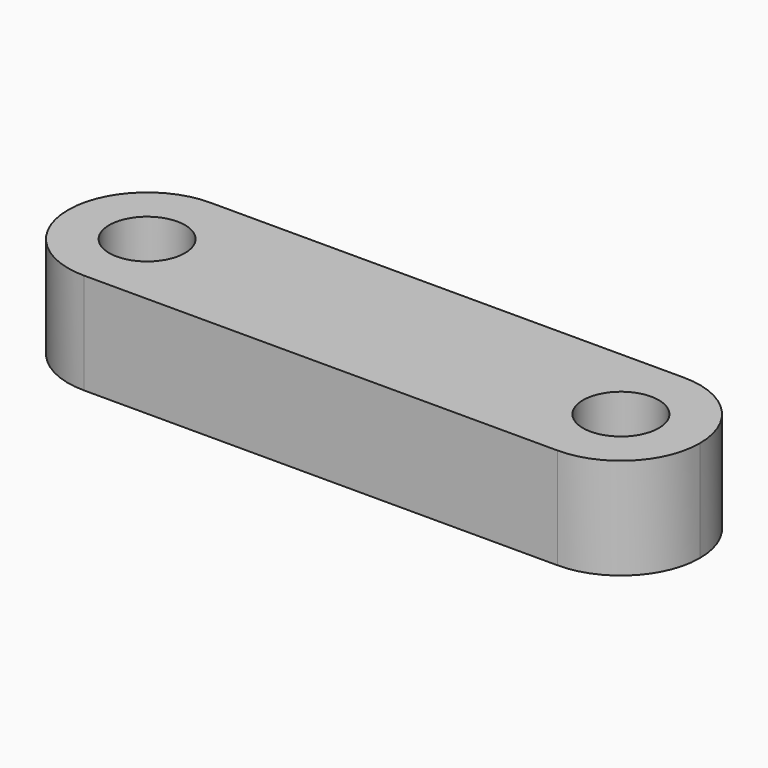
from build123d import *

# Parameters (mm, degrees)
F0_R     = 6
F1_DEPTH = 16


# Not quite as in the source:
# - a feature names something its author has since deleted; it is built from what else it names


with BuildPart() as f1:
    # F0 (on Top) → F1 (new body)
    with BuildSketch(Plane.XY):
        with BuildLine():
            Line((75, 12.5), (0, 12.5))
            ThreePointArc((0, 12.5), (8.8388347648, 8.8388347648), (12.5, 0))
            ThreePointArc((12.5, 0), (8.8388347648, -8.8388347648), (0, -12.5))
            Line((0, -12.5), (75, -12.5))
            ThreePointArc((75, -12.5), (62.5, 0), (75, 12.5))
        make_face()
        with BuildLine():
            ThreePointArc((12.5, 0), (8.8388347648, 8.8388347648), (0, 12.5))
            ThreePointArc((0, 12.5), (-8.8388347648, 8.8388347648), (-12.5, 0))
            ThreePointArc((-12.5, 0), (-8.8388347648, -8.8388347648), (0, -12.5))
            ThreePointArc((0, -12.5), (8.8388347648, -8.8388347648), (12.5, 0))
        make_face()
        Circle(F0_R, mode=Mode.SUBTRACT)
        with BuildLine():
            ThreePointArc((87.5, 0), (83.8388347648, 8.8388347648), (75, 12.5))
            ThreePointArc((75, 12.5), (62.5, 0), (75, -12.5))
            ThreePointArc((75, -12.5), (83.8388347648, -8.8388347648), (87.5, 0))
        make_face()
        with Locations((75, 0)):
            Circle(F0_R, mode=Mode.SUBTRACT)
    extrude(amount=F1_DEPTH)


solid = f1.part
